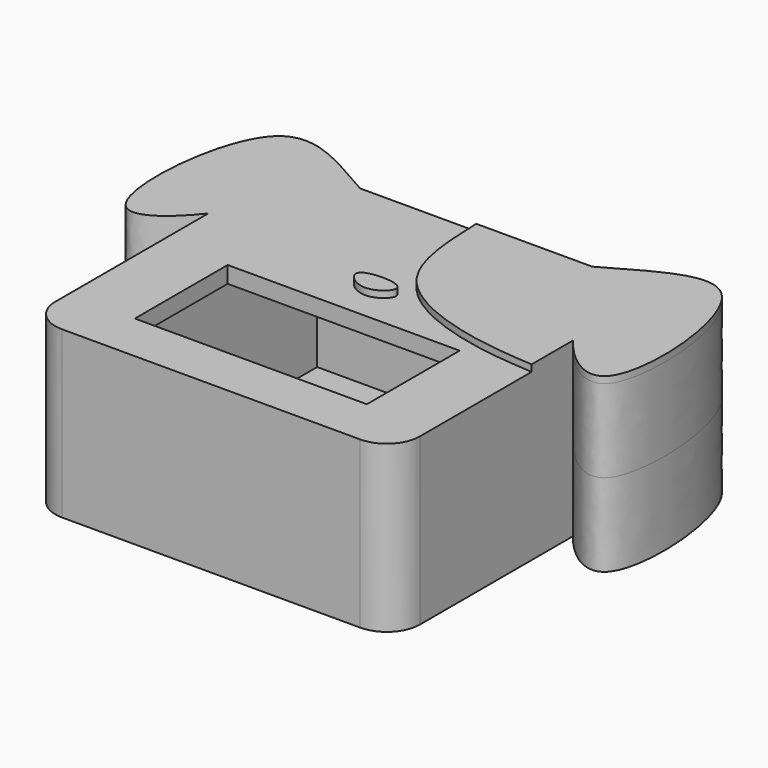
from build123d import *

# Parameters (mm, degrees)
F3_DEPTH  = 12.5
F0_W      = 40
F0_H      = 40
F4_DEPTH  = 10
F1_W      = 35
F1_H      = 17.5
F5_DEPTH  = 12.5
F7_DEPTH  = 1
F9_DEPTH  = 3.75
F10_DEPTH = 1
F11_R     = 5


with BuildPart() as f3:
    # F2 (on Top) → F3 (new body, symmetric)
    with BuildSketch(Plane.XY):
        with BuildLine():
            Line((-27.5, -25), (27.5, -25))
            Line((27.5, -25), (27.5, 8.864674))
            add(Edge.make_bspline(
                [(17.5, 25), (24.018569, 28.657121), (37.404095, 37.904593), (40.392515, -2.540506), (30.43462, 5.06004), (27.5, 8.864674)],
                knots=[0, 0, 0, 0, 0.33524, 0.742186, 1, 1, 1, 1], degree=3))
            Line((17.5, 25), (-17.5, 25))
            add(Edge.make_bspline(
                [(-17.5, 25), (-24.018569, 28.657121), (-37.404095, 37.904593), (-40.392515, -2.540506), (-30.43462, 5.06004), (-27.5, 8.864674)],
                knots=[0, 0, 0, 0, 0.33524, 0.742186, 1, 1, 1, 1], degree=3))
            Line((-27.5, 8.864674), (-27.5, -25))
        make_face()
    extrude(amount=F3_DEPTH, both=True)

    # F0 (on Top) → F4 (cut, symmetric)
    with BuildSketch(Plane.XY):
        Rectangle(F0_W, F0_H)
    extrude(amount=F4_DEPTH, both=True, mode=Mode.SUBTRACT)

    # F1 (on Top) → F5 (cut, symmetric)
    with BuildSketch(Plane.XY):
        with Locations((0, -8.75)):
            Rectangle(F1_W, F1_H)
    extrude(amount=F5_DEPTH, both=True, mode=Mode.SUBTRACT)

    # F8 (on Top) → F9 (join, symmetric)
    with BuildSketch(Plane.XY):
        with BuildLine():
            ThreePointArc((3, 25), (2.12132, 27.12132), (0, 28))
            ThreePointArc((0, 28), (-2.12132, 27.12132), (-3, 25))
            Line((-3, 25), (-2, 25))
            ThreePointArc((-2, 25), (-1.414214, 26.414214), (0, 27))
            ThreePointArc((0, 27), (1.414214, 26.414214), (2, 25))
            Line((2, 25), (3, 25))
        make_face()
    extrude(amount=F9_DEPTH, both=True)

    # F6 (on face) → F10 (join)
    with BuildSketch(Plane.XY.offset(12.5)):
        with BuildLine():
            Line((17.5, 25), (0, 25))
            add(Edge.make_bspline(
                [(0, 25), (0.20855, 19.228158), (0.618187, 7.890985), (16.3991, 1.837379), (23.969274, 1.314665), (27.5, 1.070871)],
                knots=[0, 0, 0, 0, 0.356251, 0.699756, 1, 1, 1, 1], degree=3))
            Line((27.5, 1.070871), (27.5, 8.864674))
            add(Edge.make_bspline(
                [(17.5, 25), (24.018569, 28.657121), (37.404095, 37.904593), (40.392515, -2.540506), (30.43462, 5.06004), (27.5, 8.864674)],
                knots=[0, 0, 0, 0, 0.33524, 0.742186, 1, 1, 1, 1], degree=3))
        make_face()
    extrude(amount=F10_DEPTH)

    # F11
    f11_edges = [f3.edges().sort_by_distance(p)[0] for p in [
        (27.5, -25, 0),
        (-27.5, -25, 0),
    ]]
    fillet(f11_edges, radius=F11_R)


with BuildPart() as f7:
    # F6 (on face) → F7 (new body)
    with BuildSketch(Plane.XY.offset(12.5)):
        with BuildLine():
            add(Edge.make_bspline(
                [(0, 4.103883), (1.749359, 4.119554), (5.573094, 7.708203), (-5.834426, 7.692321), (-1.778589, 4.08795), (0, 4.103883)],
                knots=[0, 0, 0, 0, 0.306768, 0.688106, 1, 1, 1, 1], degree=3))
        make_face()
    extrude(amount=F7_DEPTH)


solid = Compound([f3.part, f7.part])
